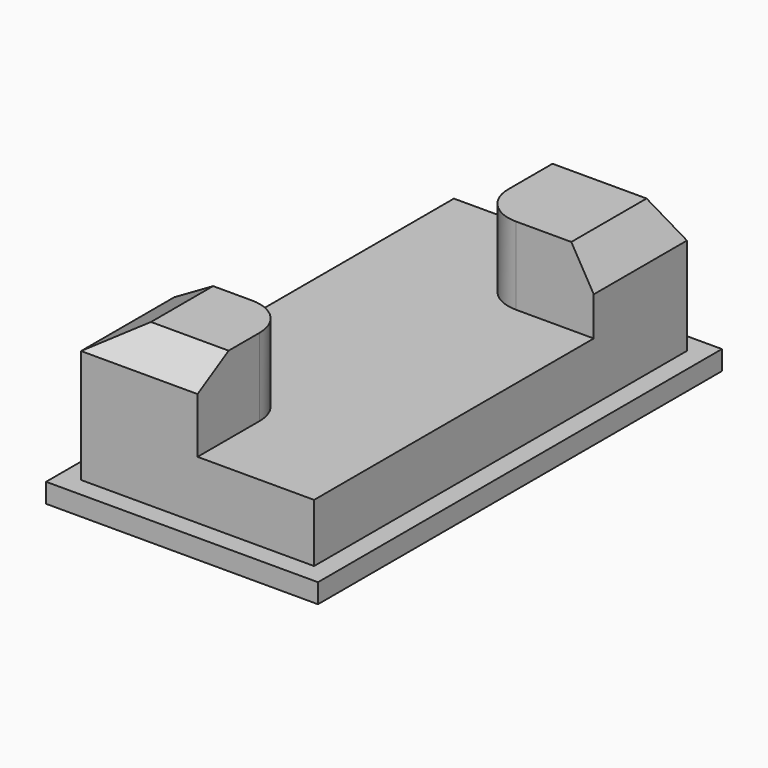
from build123d import *

# Parameters (mm, degrees)
F0_W        = 88.9
F0_H        = 165.1
F1_DEPTH    = 6.35
F2_DEPTH    = 25.4
F3_DEPTH    = 50.8
F4_C1_SIZE2 = 7.3323484187
F4_C1_SIZE  = 12.7
F4_C2_SIZE2 = 12.7
F4_C2_SIZE  = 7.3323484187
F4_C3_SIZE2 = 12.7
F4_C3_SIZE  = 7.3323484187
F4_C4_SIZE2 = 7.3323484187
F4_C4_SIZE  = 12.7


with BuildPart() as f1:
    # F0 (on Top) → F1 (new body)
    with BuildSketch(Plane.XY):
        Rectangle(F0_W, F0_H)
        Polygon((38.1, 38.1), (38.1, -76.2), (0, -76.2), (-38.1, -76.2), (-38.1, -38.1), (-38.1, 76.2), (0, 76.2), (38.1, 76.2), align=None, mode=Mode.SUBTRACT)
    extrude(amount=F1_DEPTH)

    # F0 (on Top) → F2 (join)
    with BuildSketch(Plane.XY):
        with BuildLine():
            Line((0, -76.2), (38.1, -76.2))
            Line((38.1, -76.2), (38.1, 38.1))
            Line((38.1, 38.1), (12.7, 38.1))
            ThreePointArc((12.7, 38.1), (3.7197438789, 41.8197438789), (0, 50.8))
            Line((0, 50.8), (0, 76.2))
            Line((0, 76.2), (-38.1, 76.2))
            Line((-38.1, 76.2), (-38.1, -38.1))
            Line((-38.1, -38.1), (-12.7, -38.1))
            ThreePointArc((-12.7, -38.1), (-3.7197438789, -41.8197438789), (0, -50.8))
            Line((0, -50.8), (0, -76.2))
        make_face()
    extrude(amount=F2_DEPTH)

    # F0 (on Top) → F3 (join)
    with BuildSketch(Plane.XY):
        with BuildLine():
            Line((-38.1, -76.2), (0, -76.2))
            Line((0, -76.2), (0, -50.8))
            ThreePointArc((0, -50.8), (-3.7197438789, -41.8197438789), (-12.7, -38.1))
            Line((-12.7, -38.1), (-38.1, -38.1))
            Line((-38.1, -38.1), (-38.1, -76.2))
        make_face()
        with BuildLine():
            Line((12.7, 38.1), (38.1, 38.1))
            Line((38.1, 38.1), (38.1, 76.2))
            Line((38.1, 76.2), (0, 76.2))
            Line((0, 76.2), (0, 50.8))
            ThreePointArc((0, 50.8), (3.7197438789, 41.8197438789), (12.7, 38.1))
        make_face()
    extrude(amount=F3_DEPTH)

    # F4: chamfer of 12.7 x 7.3323484187 on 4 edges, made by hand

    # F4_c1
    f4_c1_edges = [f1.edges().sort_by_distance(p)[0] for p in [
        (19.05, 76.2, 50.8),
    ]]
    f4_c1_side = f1.faces().sort_by_distance((19.05, 76.2, 50.6533530316))[0]
    chamfer(f4_c1_edges, length=F4_C1_SIZE, length2=F4_C1_SIZE2, reference=f4_c1_side)

    # F4_c2
    f4_c2_edges = [f1.edges().sort_by_distance(p)[0] for p in [
        (-19.05, -76.2, 50.8),
    ]]
    f4_c2_side = f1.faces().sort_by_distance((-19.05, -76.2, 50.6533530316))[0]
    chamfer(f4_c2_edges, length=F4_C2_SIZE, length2=F4_C2_SIZE2, reference=f4_c2_side)

    # F4_c3
    f4_c3_edges = [f1.edges().sort_by_distance(p)[0] for p in [
        (-38.1, -50.8, 50.8),
    ]]
    f4_c3_side = f1.faces().sort_by_distance((-38.1, -50.8, 50.6533530316))[0]
    chamfer(f4_c3_edges, length=F4_C3_SIZE, length2=F4_C3_SIZE2, reference=f4_c3_side)

    # F4_c4
    f4_c4_edges = [f1.edges().sort_by_distance(p)[0] for p in [
        (38.1, 53.4838257906, 50.8),
    ]]
    f4_c4_side = f1.faces().sort_by_distance((38.1, 53.4838257906, 50.6533530316))[0]
    chamfer(f4_c4_edges, length=F4_C4_SIZE, length2=F4_C4_SIZE2, reference=f4_c4_side)


solid = f1.part
